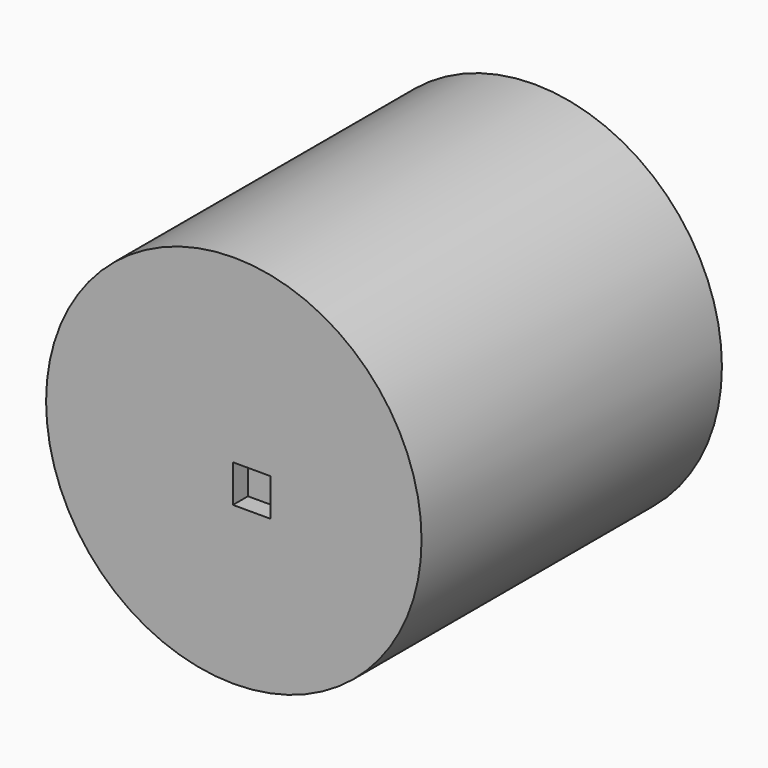
from build123d import *

# Parameters (mm, degrees)
F0_R          = 254
F1_DEPTH      = 508
F2_W          = 50.8
F2_H          = 50.8
F3_DEPTH      = 25.4
F3_DEPTH_BACK = 1134


# Not quite as in the source:
# - an extrude ends at something that could not be found from the text; its depth is read off the source's solid


with BuildPart() as f1:
    # F0 (on Front) → F1 (new body)
    with BuildSketch(Plane.XZ):
        with Locations((0, 1.6020847252)):
            Circle(F0_R)
    extrude(amount=F1_DEPTH)

    # F2 (on face) → F3 (cut, two sides)
    with BuildSketch(Plane.XZ.offset(508)) as f3_sk:
        with Locations((24.2332161129, -14.1495072007)):
            Rectangle(F2_W, F2_H)
    extrude(amount=-F3_DEPTH, mode=Mode.SUBTRACT)
    extrude(f3_sk.sketch, amount=F3_DEPTH_BACK, mode=Mode.SUBTRACT)


solid = f1.part
